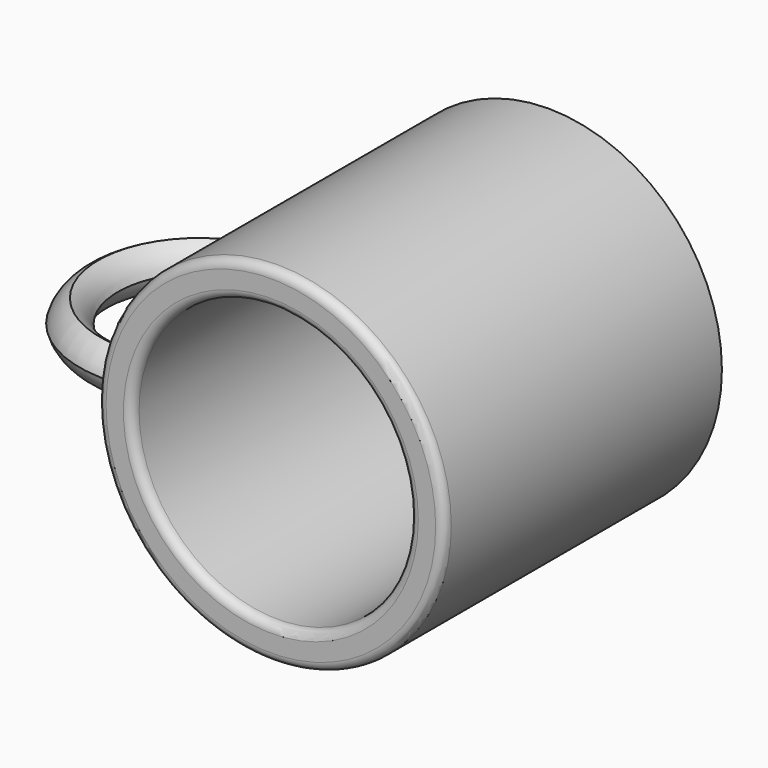
from build123d import *

# Parameters (mm, degrees)
F0_R        = 25.4
F1_DEPTH    = 50.8
F2_T        = -5.08
F3_R        = 1.27
F5_DEPTH    = 3.81
F6_W        = 1.8350626505
F6_H        = 35.56
F7_DEPTH    = 3.81
F8_T2_ANGLE = 305.4756287564
F8_T4_ANGLE = 305.4756287564
F8_T6_ANGLE = 272.5058510715
F8_T8_ANGLE = 272.5058510715


# Not quite as in the source:
# - a fillet or chamfer that OpenCascade refuses, or shapes differently, is made with other operations: its cross-section is extruded or revolved along the edge and cut away or added


with BuildPart() as f1:
    # F0 (on Front) → F1 (new body)
    with BuildSketch(Plane.XZ):
        Circle(F0_R)
    extrude(amount=F1_DEPTH)

    # F2
    f2_openings = [f1.faces().sort_by_distance(p)[0] for p in [
        (0, -50.8, 0),
    ]]
    offset(amount=F2_T, openings=f2_openings)

    # F3
    f3_edges = [f1.edges().sort_by_distance(p)[0] for p in [
        (-25.4, -50.8, 0),
        (-20.32, -50.8, 0),
    ]]
    fillet(f3_edges, radius=F3_R)


with BuildPart() as f5:
    # F4 (on Top) → F5 (new body, symmetric)
    with BuildSketch(Plane.XY):
        with BuildLine():
            ThreePointArc((-26.8851481378, -40.5866503716), (-40.3914383995, -28.1052119099), (-26.8851481378, -15.6237734482))
            Line((-26.8851481378, -15.6237734482), (-26.8851481378, -10.7935341075))
            ThreePointArc((-26.8851481378, -10.7935341075), (-46.0874012872, -28.3924848773), (-26.8851481378, -45.991435647))
            Line((-26.8851481378, -45.991435647), (-26.8851481378, -40.5866503716))
        make_face()
    extrude(amount=F5_DEPTH, both=True)

    # F8: fillet of radius 5.08 on 4 edges, made by hand

    # F8_s1 → F8_t2 (revolve, cut)
    with BuildSketch(Plane(origin=(-17.2918796722, -33.5567244349, 0), x_dir=(0, 0, 1), z_dir=(0.4580629802, 0.8889197411, 0))):
        with BuildLine():
            ThreePointArc((1.27, 0.61909191), (-2.3221024484, 2.1069894616), (-3.81, 5.69909191))
            Line((-3.81, 5.69909191), (-3.81, 0.61909191))
            Line((-3.81, 0.61909191), (1.27, 0.61909191))
        make_face()
    revolve(axis=Axis((-27.8711172694, -28.1052119099, -3.81), (0, 0, -1)), revolution_arc=F8_T2_ANGLE, mode=Mode.SUBTRACT)

    # F8_s3 → F8_t4 (revolve, cut)
    with BuildSketch(Plane(origin=(-17.2918796722, -33.5567244349, 0), x_dir=(0, 0, 1), z_dir=(0.4580629802, 0.8889197411, 0))):
        with BuildLine():
            ThreePointArc((3.81, 5.69909191), (2.3221024484, 2.1069894616), (-1.27, 0.61909191))
            Line((-1.27, 0.61909191), (3.81, 0.61909191))
            Line((3.81, 0.61909191), (3.81, 5.69909191))
        make_face()
    revolve(axis=Axis((-27.8711172694, -28.1052119099, 3.81), (0, 0, -1)), revolution_arc=F8_T4_ANGLE, mode=Mode.SUBTRACT)

    # F8_s5 → F8_t6 (revolve, cut)
    with BuildSketch(Plane(origin=(0.5932237272, -0.6197529366, 0), x_dir=(0, 0, 1), z_dir=(0.6914761708, -0.7223992699, 0))):
        with BuildLine():
            ThreePointArc((1.27, 22.498524229), (-2.3221024484, 23.9864217805), (-3.81, 27.578524229))
            Line((-3.81, 27.578524229), (-3.81, 22.498524229))
            Line((-3.81, 22.498524229), (1.27, 22.498524229))
        make_face()
    revolve(axis=Axis((-28.4215162233, -28.3924848773, -3.81), (0, 0, 1)), revolution_arc=F8_T6_ANGLE, mode=Mode.SUBTRACT)

    # F8_s7 → F8_t8 (revolve, cut)
    with BuildSketch(Plane(origin=(0.5932237272, -0.6197529366, 0), x_dir=(0, 0, 1), z_dir=(0.6914761708, -0.7223992699, 0))):
        with BuildLine():
            ThreePointArc((-1.27, 22.498524229), (2.3221024484, 23.9864217805), (3.81, 27.578524229))
            Line((3.81, 27.578524229), (3.81, 22.498524229))
            Line((3.81, 22.498524229), (-1.27, 22.498524229))
        make_face()
    revolve(axis=Axis((-28.4215162233, -28.3924848773, 3.81), (0, 0, 1)), revolution_arc=F8_T8_ANGLE, mode=Mode.SUBTRACT)


with BuildPart() as f7:
    # F6 (on Top) → F7 (new body, symmetric)
    with BuildSketch(Plane.XY):
        with Locations((-25.9598139673, -28.4927496687)):
            Rectangle(F6_W, F6_H)
    extrude(amount=F7_DEPTH, both=True)


solid = Compound([f1.part, f5.part, f7.part])
